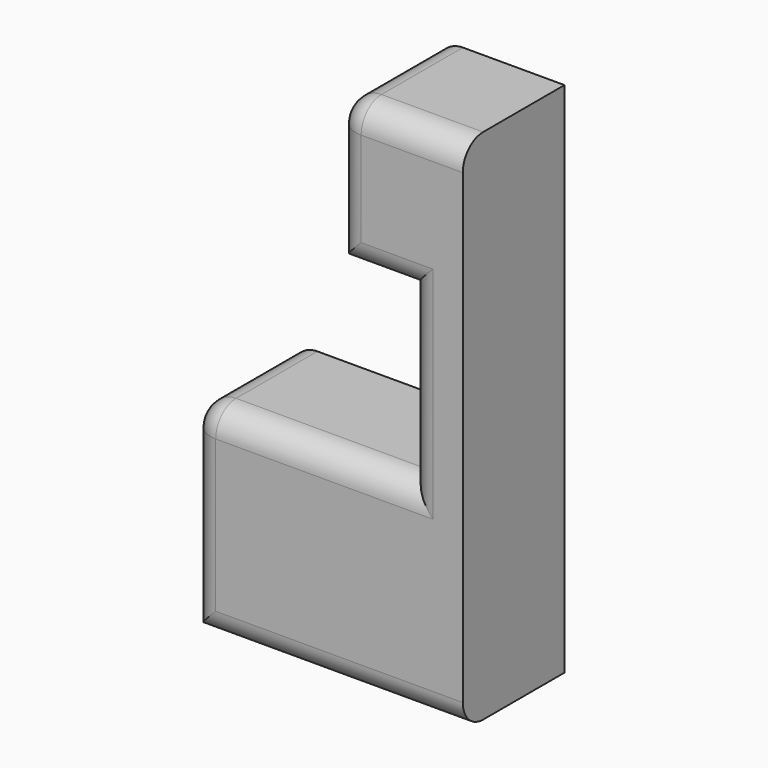
from build123d import *

# Parameters (mm, degrees)
F1_DEPTH    = 25.4
F2_R        = 5.08
F3_R        = 5.08
F4_T1_DEPTH = 33.02
F4_S5_W     = 5.08
F4_S5_H     = 5.08
F4_T6_DEPTH = 5.08


# Not quite as in the source:
# - a fillet or chamfer that OpenCascade refuses, or shapes differently, is made with other operations: its cross-section is extruded or revolved along the edge and cut away or added


with BuildPart() as f1:
    # F0 (on Front) → F1 (new body)
    with BuildSketch(Plane.XZ):
        Polygon((0, -50.5684018135), (0, 52.7750141919), (-25.3761447966, 52.7750141919), (-25.3761447966, 23.721171543), (-11.0331093892, 23.721171543), (-11.0331093892, -10.1136825979), (-54.4299855828, -10.1136825979), (-54.4299855828, -50.5684018135), align=None)
    extrude(amount=F1_DEPTH)

    # F2
    f2_edges = [f1.edges().sort_by_distance(p)[0] for p in [
        (-12.688072, -25.4, 52.775014),
    ]]
    fillet(f2_edges, radius=F2_R)

    # F3
    f3_edges = [f1.edges().sort_by_distance(p)[0] for p in [
        (-27.214993, -25.4, -50.568402),
        (-54.429986, -25.4, -30.341042),
        (-32.731547, -25.4, -10.113683),
        (-11.033109, -25.4, 6.803744),
        (-25.376145, -25.4, 35.708093),
        (-18.204627, -25.4, 23.721172),
    ]]
    fillet(f3_edges, radius=F3_R)

    # F4: fillet of radius 5.08 on 1 edges, made by hand

    # F4_s2 → F4_t1 (cut)
    with BuildSketch(Plane.XZ.offset(-12.7)):
        with BuildLine():
            ThreePointArc((-54.4299855828, -15.1936825979), (-52.9420880313, -11.6015801494), (-49.3499855828, -10.1136825979))
            Line((-49.3499855828, -10.1136825979), (-54.4299855828, -10.1136825979))
            Line((-54.4299855828, -10.1136825979), (-54.4299855828, -15.1936825979))
        make_face()
    extrude(amount=F4_T1_DEPTH, mode=Mode.SUBTRACT)


with BuildPart() as f4_tool4:
    # F4_s5 → F4_t6 (new body)
    with BuildSketch(Plane.YZ.offset(-49.3499855828)):
        with Locations((-22.86, -12.6536825979)):
            Rectangle(F4_S5_W, F4_S5_H)
    extrude(amount=-F4_T6_DEPTH)

    # F4_s7 → F4_t8 (revolve, cut)
    with BuildSketch(Plane(origin=(-49.3499855828, -20.32, -15.1936825979), x_dir=(0, 0.7071067812, -0.7071067812), z_dir=(0, 0.7071067812, 0.7071067812))):
        with BuildLine():
            ThreePointArc((0, -5.08), (5.08, 0), (0, 5.08))
            Line((0, 5.08), (0, -5.08))
        make_face()
    revolve(axis=Axis((-49.3499855828, -20.32, -15.1936825979), (-1, 0, 0)), mode=Mode.SUBTRACT)


with BuildPart() as f1_1:
    add(f1.part)

    # F4_t3: cut F4_tool4
    add(f4_tool4.part, mode=Mode.SUBTRACT)


solid = f1_1.part
